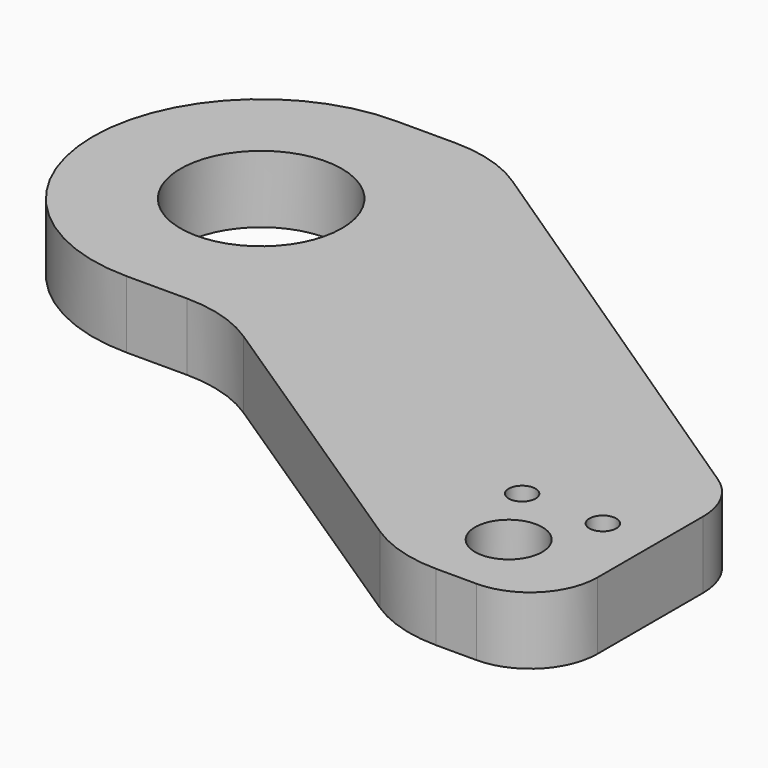
from build123d import *

# Parameters (mm, degrees)
F0_R     = 2
F0_R_2   = 5
F0_R_3   = 12
F1_DEPTH = 10
F2_R     = 24.99999
F3_R     = 10
F4_R     = 20


# Not quite as in the source:
# - a fillet or chamfer is up to 0.001 mm smaller than in the source, because OpenCascade refuses the exact size


with BuildPart() as f1:
    # F0 (on Top) → F1 (new body)
    with BuildSketch(Plane.XY):
        Polygon((-26.9614594782, 50), (-66.9614594782, 50), (-66.9614594782, 0), (-26.9614594782, 0), (26.0385405218, -35), (48.0385405218, -35), (48.0385405218, 0), align=None)
        with Locations((28.0385405218, -14)):
            Circle(F0_R, mode=Mode.SUBTRACT)
        with Locations((34.0385405218, -24)):
            Circle(F0_R_2, mode=Mode.SUBTRACT)
        with Locations((40.0385405218, -14)):
            Circle(F0_R, mode=Mode.SUBTRACT)
        with Locations((-41.9614594782, 25)):
            Circle(F0_R_3, mode=Mode.SUBTRACT)
    extrude(amount=F1_DEPTH)

    # F2 (radius 25 in the source; OpenCascade refuses exactly that, so slightly less here)
    f2_edges = [f1.edges().sort_by_distance(p)[0] for p in [
        (-66.961459, 50, 5),
        (-66.961459, 0, 5),
    ]]
    fillet(f2_edges, radius=F2_R)

    # F3
    f3_edges = [f1.edges().sort_by_distance(p)[0] for p in [
        (48.038541, -35, 5),
        (48.038541, 0, 5),
    ]]
    fillet(f3_edges, radius=F3_R)

    # F4
    f4_edges = [f1.edges().sort_by_distance(p)[0] for p in [
        (-26.961459, 50, 5),
        (-26.961459, 0, 5),
        (26.038541, -35, 5),
    ]]
    fillet(f4_edges, radius=F4_R)


solid = f1.part
